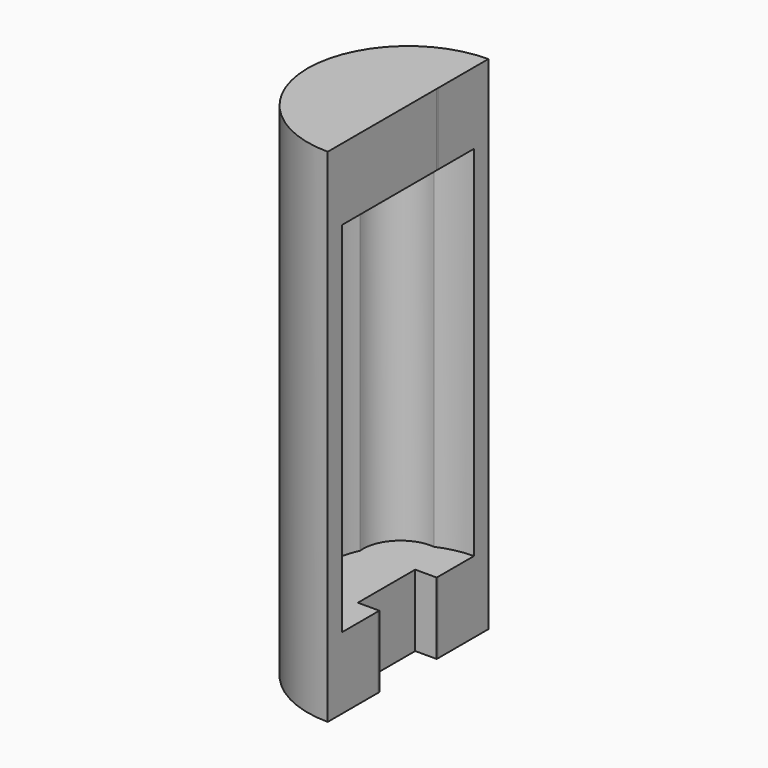
from build123d import *

# Parameters (mm, degrees)
F1_DEPTH = 10
F2_DEPTH = 50
F3_DEPTH = 10
F4_START = 50
F4_DEPTH = 10


# Not quite as in the source:
# - a feature names something its author has since deleted; it is built from what else it names


with BuildPart() as f1:
    # F0 (on Top) → F1 (new body)
    with BuildSketch(Plane.XY):
        with BuildLine():
            Line((0, 11.5), (0, 14))
            ThreePointArc((0, 14), (-14, 0), (0, -14))
            Line((0, -14), (0, -11.5))
            ThreePointArc((0, -11.5), (-2.4269719101, -11.2409878279), (-4.7446194261, -10.4756186692))
            ThreePointArc((-4.7446194261, -10.4756186692), (-8.9623106012, -8.9623106012), (-10.4756186692, -4.7446194261))
            ThreePointArc((-10.4756186692, -4.7446194261), (-11.5, 0), (-10.4756186692, 4.7446194261))
            ThreePointArc((-10.4756186692, 4.7446194261), (-8.9623106012, 8.9623106012), (-4.7446194261, 10.4756186692))
            ThreePointArc((-4.7446194261, 10.4756186692), (-2.4269719101, 11.2409878279), (0, 11.5))
        make_face()
        with BuildLine():
            ThreePointArc((-4.7446194261, -10.4756186692), (-2.4269719101, -11.2409878279), (0, -11.5))
            Line((0, -11.5), (0, -9))
            Line((0, -9), (0, -5.25))
            ThreePointArc((0, -5.25), (-1.3631151282, -8.7791112186), (-4.7446194261, -10.4756186692))
        make_face()
        with BuildLine():
            Line((-5.25, -5.25), (0, -5.25))
            ThreePointArc((0, -5.25), (-0.001489151, -5.124964534), (-0.0059557591, -5))
            Line((-0.0059557591, -5), (-3, -5))
            Line((-3, -5), (-3, -0.5065835097))
            ThreePointArc((-3, -0.5065835097), (-4.0968383837, -0.1282114172), (-5.2499999999, 0))
            Line((-5.25, 0), (-5.25, -5.25))
        make_face()
        with BuildLine():
            ThreePointArc((-10.4756186692, -4.7446194261), (-8.1317279836, -8.1317279836), (-4.7446194261, -10.4756186692))
            ThreePointArc((-4.7446194261, -10.4756186692), (-1.3631151282, -8.7791112186), (0, -5.25))
            Line((0, -5.25), (-5.25, -5.25))
            Line((-5.25, -5.25), (-5.25, 0))
            ThreePointArc((-5.2499999999, 0), (-8.7791112186, -1.3631151282), (-10.4756186692, -4.7446194261))
        make_face()
        with BuildLine():
            ThreePointArc((-5.2499999999, 0), (-8.7791112186, 1.3631151282), (-10.4756186692, 4.7446194261))
            ThreePointArc((-10.4756186692, 4.7446194261), (-11.5, 0), (-10.4756186692, -4.7446194261))
            ThreePointArc((-10.4756186692, -4.7446194261), (-8.7791112186, -1.3631151282), (-5.2499999999, 0))
        make_face()
        with BuildLine():
            ThreePointArc((-3, 0.5065835097), (-4.0968383837, 0.1282114172), (-5.2499999999, 0))
            ThreePointArc((-5.2499999999, 0), (-4.0968383837, -0.1282114172), (-3, -0.5065835097))
            Line((-3, -0.5065835097), (-3, 0.5065835097))
        make_face()
        with BuildLine():
            ThreePointArc((0, 5.25), (-1.3631151282, 8.7791112186), (-4.7446194261, 10.4756186692))
            ThreePointArc((-4.7446194261, 10.4756186692), (-8.1317279836, 8.1317279836), (-10.4756186692, 4.7446194261))
            ThreePointArc((-10.4756186692, 4.7446194261), (-8.7791112186, 1.3631151282), (-5.2499999999, 0))
            Line((-5.25, 0), (-5.25, 5.25))
            Line((-5.25, 5.25), (0, 5.25))
        make_face()
        with BuildLine():
            Line((0, 9), (0, 11.5))
            ThreePointArc((0, 11.5), (-2.4269719101, 11.2409878279), (-4.7446194261, 10.4756186692))
            ThreePointArc((-4.7446194261, 10.4756186692), (-1.3631151282, 8.7791112186), (0, 5.25))
            Line((0, 5.25), (0, 6))
            Line((0, 6), (0, 9))
        make_face()
        with BuildLine():
            ThreePointArc((-10.4756186692, 4.7446194261), (-8.1317279836, 8.1317279836), (-4.7446194261, 10.4756186692))
            ThreePointArc((-4.7446194261, 10.4756186692), (-8.9623106012, 8.9623106012), (-10.4756186692, 4.7446194261))
        make_face()
        with BuildLine():
            ThreePointArc((-10.4756186692, -4.7446194261), (-8.9623106012, -8.9623106012), (-4.7446194261, -10.4756186692))
            ThreePointArc((-4.7446194261, -10.4756186692), (-8.1317279836, -8.1317279836), (-10.4756186692, -4.7446194261))
        make_face()
        with BuildLine():
            ThreePointArc((-0.0059557591, 5), (-0.001489151, 5.124964534), (0, 5.25))
            Line((0, 5.25), (-5.25, 5.25))
            Line((-5.25, 5.25), (-5.25, 0))
            ThreePointArc((-5.2499999999, 0), (-4.0968383837, 0.1282114172), (-3, 0.5065835097))
            Line((-3, 0.5065835097), (-3, 5))
            Line((-3, 5), (-0.0059557591, 5))
        make_face()
    extrude(amount=-F1_DEPTH)

    # F0 (on Top) → F2 (join)
    with BuildSketch(Plane.XY):
        with BuildLine():
            Line((0, 11.5), (0, 14))
            ThreePointArc((0, 14), (-14, 0), (0, -14))
            Line((0, -14), (0, -11.5))
            ThreePointArc((0, -11.5), (-2.4269719101, -11.2409878279), (-4.7446194261, -10.4756186692))
            ThreePointArc((-4.7446194261, -10.4756186692), (-8.9623106012, -8.9623106012), (-10.4756186692, -4.7446194261))
            ThreePointArc((-10.4756186692, -4.7446194261), (-11.5, 0), (-10.4756186692, 4.7446194261))
            ThreePointArc((-10.4756186692, 4.7446194261), (-8.9623106012, 8.9623106012), (-4.7446194261, 10.4756186692))
            ThreePointArc((-4.7446194261, 10.4756186692), (-2.4269719101, 11.2409878279), (0, 11.5))
        make_face()
    extrude(amount=F2_DEPTH)

    # F3 (add): a face of the model
    f3_faces = [f1.faces().sort_by_distance(p)[0] for p in [
        (-2.4930382043, 11.5469865939, 50),
    ]]
    extrude(f3_faces, amount=F3_DEPTH)

    # F0 (on Top) → F4 (join)
    with BuildSketch(Plane.XY.offset(F4_START)):
        with BuildLine():
            Line((0, 9), (0, 11.5))
            ThreePointArc((0, 11.5), (-2.4269719101, 11.2409878279), (-4.7446194261, 10.4756186692))
            ThreePointArc((-4.7446194261, 10.4756186692), (-1.3631151282, 8.7791112186), (0, 5.25))
            Line((0, 5.25), (0, 6))
            Line((0, 6), (0, 9))
        make_face()
        with BuildLine():
            ThreePointArc((-4.7446194261, -10.4756186692), (-2.4269719101, -11.2409878279), (0, -11.5))
            Line((0, -11.5), (0, -9))
            Line((0, -9), (0, -5.25))
            ThreePointArc((0, -5.25), (-1.3631151282, -8.7791112186), (-4.7446194261, -10.4756186692))
        make_face()
        with BuildLine():
            ThreePointArc((0, 5.25), (-1.3631151282, 8.7791112186), (-4.7446194261, 10.4756186692))
            ThreePointArc((-4.7446194261, 10.4756186692), (-8.1317279836, 8.1317279836), (-10.4756186692, 4.7446194261))
            ThreePointArc((-10.4756186692, 4.7446194261), (-8.7791112186, 1.3631151282), (-5.2499999999, 0))
            Line((-5.25, 0), (-5.25, 5.25))
            Line((-5.25, 5.25), (0, 5.25))
        make_face()
        with BuildLine():
            ThreePointArc((-10.4756186692, 4.7446194261), (-8.1317279836, 8.1317279836), (-4.7446194261, 10.4756186692))
            ThreePointArc((-4.7446194261, 10.4756186692), (-8.9623106012, 8.9623106012), (-10.4756186692, 4.7446194261))
        make_face()
        with BuildLine():
            ThreePointArc((-10.4756186692, -4.7446194261), (-8.9623106012, -8.9623106012), (-4.7446194261, -10.4756186692))
            ThreePointArc((-4.7446194261, -10.4756186692), (-8.1317279836, -8.1317279836), (-10.4756186692, -4.7446194261))
        make_face()
        with BuildLine():
            ThreePointArc((-10.4756186692, -4.7446194261), (-8.1317279836, -8.1317279836), (-4.7446194261, -10.4756186692))
            ThreePointArc((-4.7446194261, -10.4756186692), (-1.3631151282, -8.7791112186), (0, -5.25))
            Line((0, -5.25), (-5.25, -5.25))
            Line((-5.25, -5.25), (-5.25, 0))
            ThreePointArc((-5.2499999999, 0), (-8.7791112186, -1.3631151282), (-10.4756186692, -4.7446194261))
        make_face()
        with BuildLine():
            ThreePointArc((-5.2499999999, 0), (-8.7791112186, 1.3631151282), (-10.4756186692, 4.7446194261))
            ThreePointArc((-10.4756186692, 4.7446194261), (-11.5, 0), (-10.4756186692, -4.7446194261))
            ThreePointArc((-10.4756186692, -4.7446194261), (-8.7791112186, -1.3631151282), (-5.2499999999, 0))
        make_face()
        with BuildLine():
            ThreePointArc((-0.0059557591, 5), (-0.001489151, 5.124964534), (0, 5.25))
            Line((0, 5.25), (-5.25, 5.25))
            Line((-5.25, 5.25), (-5.25, 0))
            ThreePointArc((-5.2499999999, 0), (-4.0968383837, 0.1282114172), (-3, 0.5065835097))
            Line((-3, 0.5065835097), (-3, 5))
            Line((-3, 5), (-0.0059557591, 5))
        make_face()
        with BuildLine():
            ThreePointArc((-0.0059557591, -5), (-0.001489151, -5.124964534), (0, -5.25))
            Line((0, -5.25), (0, -5))
            Line((0, -5), (-0.0059557591, -5))
        make_face()
        with BuildLine():
            Line((-5.25, -5.25), (0, -5.25))
            ThreePointArc((0, -5.25), (-0.001489151, -5.124964534), (-0.0059557591, -5))
            Line((-0.0059557591, -5), (-3, -5))
            Line((-3, -5), (-3, -0.5065835097))
            ThreePointArc((-3, -0.5065835097), (-4.0968383837, -0.1282114172), (-5.2499999999, 0))
            Line((-5.25, 0), (-5.25, -5.25))
        make_face()
        with BuildLine():
            ThreePointArc((-3, 0.5065835097), (-4.0968383837, 0.1282114172), (-5.2499999999, 0))
            ThreePointArc((-5.2499999999, 0), (-4.0968383837, -0.1282114172), (-3, -0.5065835097))
            Line((-3, -0.5065835097), (-3, 0.5065835097))
        make_face()
        with BuildLine():
            Line((0, 0), (0, 5))
            Line((0, 5), (-0.0059557591, 5))
            ThreePointArc((-0.0059557591, 5), (-0.8810329928, 2.3388786885), (-3, 0.5065835097))
            Line((-3, 0.5065835097), (-3, -0.5065835097))
            ThreePointArc((-3, -0.5065835097), (-0.8810329928, -2.3388786885), (-0.0059557591, -5))
            Line((-0.0059557591, -5), (0, -5))
            Line((0, -5), (0, 0))
        make_face()
        with BuildLine():
            ThreePointArc((-3, 0.5065835097), (-0.8810329928, 2.3388786885), (-0.0059557591, 5))
            Line((-0.0059557591, 5), (-3, 5))
            Line((-3, 5), (-3, 0.5065835097))
        make_face()
        with BuildLine():
            Line((-3, -5), (-0.0059557591, -5))
            ThreePointArc((-0.0059557591, -5), (-0.8810329928, -2.3388786885), (-3, -0.5065835097))
            Line((-3, -0.5065835097), (-3, -5))
        make_face()
    extrude(amount=F4_DEPTH)


solid = f1.part
